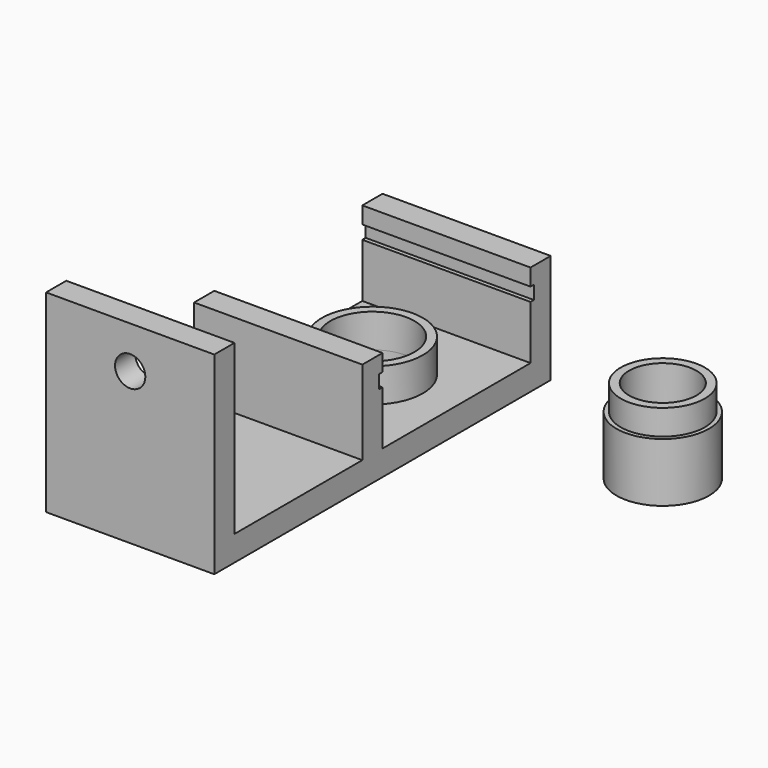
from build123d import *

# Parameters (mm, degrees)
F0_W      = 20
F0_H      = 3
F1_DEPTH  = 10
F0_R      = 6
F0_R_2    = 5
F2_DEPTH  = 4
F0_H_2    = 22
F0_H_3    = 19
F3_DEPTH  = 3
F4_W      = 20
F4_H      = 1.6
F5_DEPTH  = 0.5
F6_W      = 20
F6_H      = 1.6
F7_DEPTH  = 0.5
F8_DEPTH  = 10
F9_R      = 1.8
F10_DEPTH = 50.001
F11_R     = 5
F11_R_2   = 4
F12_DEPTH = 10
F11_R_3   = 5.5
F15_DEPTH = 7
F16_DEPTH = 10


# Not quite as in the source:
# - a feature names something its author has since deleted; it is built from what else it names
# - the program builds the solid bodies; features that only make, move or delete a surface that nothing else refers to are left out


with BuildPart() as f1:
    # F0 (on Top) → F1 (new body)
    with BuildSketch(Plane.XY):
        with Locations((0, 1.5)):
            Rectangle(F0_W, F0_H)
    extrude(amount=F1_DEPTH)



with BuildPart() as f1b:
    # F0 (on Top) → F1, piece 2 (new body)
    with BuildSketch(Plane.XY):
        with Locations((0, 23.5)):
            Rectangle(F0_W, F0_H)
    extrude(amount=F1_DEPTH)


with BuildPart() as f1c:
    # F0 (on Top) → F1, piece 3 (new body)
    with BuildSketch(Plane.XY):
        with Locations((0, 48.5)):
            Rectangle(F0_W, F0_H)
    extrude(amount=F1_DEPTH)


with BuildPart() as f2:
    # F0 (on Top) → F2 (new body)
    with BuildSketch(Plane.XY):
        with Locations((0, 36)):
            Circle(F0_R)
        with Locations((0, 36)):
            Circle(F0_R_2, mode=Mode.SUBTRACT)
    extrude(amount=F2_DEPTH)


with BuildPart() as f1_1:
    add(f1.part)

    add(f1b.part)  # F3 merges F1b

    add(f1c.part)  # F3 merges F1c

    add(f2.part)  # F3 merges F2
    # F0 (on Top) → F3 (join)
    with BuildSketch(Plane.XY):
        with Locations((0, 48.5)):
            Rectangle(F0_W, F0_H)
        with Locations((0, 36)):
            Rectangle(F0_W, F0_H_2)
        with Locations((0, 36)):
            Circle(F0_R, mode=Mode.SUBTRACT)
        with Locations((0, 36)):
            Circle(F0_R)
        with Locations((0, 36)):
            Circle(F0_R_2, mode=Mode.SUBTRACT)
        with Locations((0, 23.5)):
            Rectangle(F0_W, F0_H)
        with Locations((0, 12.5)):
            Rectangle(F0_W, F0_H_3)
        with Locations((0, 1.5)):
            Rectangle(F0_W, F0_H)
    extrude(amount=-F3_DEPTH)

    # F4 (on face) → F5 (cut)
    with BuildSketch(Plane.XZ.offset(-47)):
        with Locations((0, 7.2)):
            Rectangle(F4_W, F4_H)
    extrude(amount=-F5_DEPTH, mode=Mode.SUBTRACT)

    # F6 (on face) → F7 (cut)
    with BuildSketch(Plane(origin=(0, 25, 0), x_dir=(-1, 0, 0), z_dir=(0, 1, 0))):
        with Locations((0, 7.2)):
            Rectangle(F6_W, F6_H)
    extrude(amount=-F7_DEPTH, mode=Mode.SUBTRACT)

    # F8 (add): a face of the model
    f8_faces = [f1_1.faces().sort_by_distance(p)[0] for p in [
        (0, 1.5, 10),
    ]]
    extrude(f8_faces, amount=F8_DEPTH)

    # F9 (on Front) → F10 (cut, through all)
    with BuildSketch(Plane.XZ):
        with Locations((0, 15)):
            Circle(F9_R)
    extrude(amount=-F10_DEPTH, mode=Mode.SUBTRACT)


with BuildPart() as f12:
    # F11 (on Top) → F12 (new body)
    with BuildSketch(Plane.XY):
        with Locations((34.0979397297, 36.5335047245)):
            Circle(F11_R)
        with Locations((34.0979397297, 36.5335047245)):
            Circle(F11_R_2, mode=Mode.SUBTRACT)
    extrude(amount=F12_DEPTH)


with BuildPart() as f15:
    # F11 (on Top) → F15 (new body)
    with BuildSketch(Plane.XY):
        with Locations((34.0979397297, 36.5335047245)):
            Circle(F11_R_3)
        with Locations((34.0979397297, 36.5335047245)):
            Circle(F11_R, mode=Mode.SUBTRACT)
        with Locations((34.0979397297, 36.5335047245)):
            Circle(F11_R)
        with Locations((34.0979397297, 36.5335047245)):
            Circle(F11_R_2, mode=Mode.SUBTRACT)
    extrude(amount=F15_DEPTH)

    # F11 (on Top) → F16 (join)
    with BuildSketch(Plane.XY):
        with Locations((34.0979397297, 36.5335047245)):
            Circle(F11_R)
        with Locations((34.0979397297, 36.5335047245)):
            Circle(F11_R_2, mode=Mode.SUBTRACT)
    extrude(amount=F16_DEPTH)


solid = Compound([f1_1.part, f15.part])
